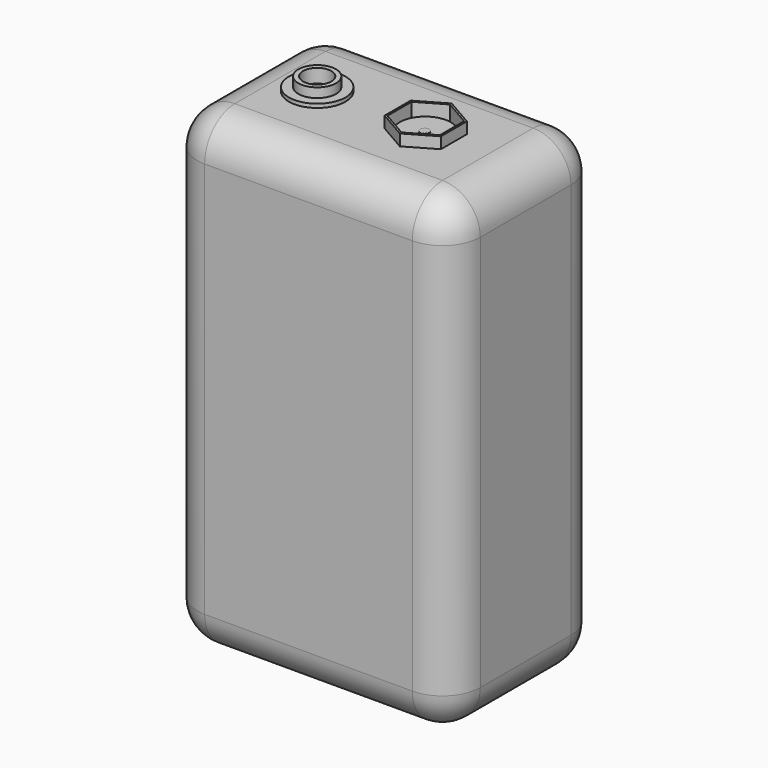
from build123d import *

# Parameters (mm, degrees)
F0_W      = 38.1
F0_H      = 63.5
F1_DEPTH  = 25.4
F2_R      = 5.08
F3_R      = 3.81
F4_DEPTH  = 0.508
F5_R      = 2.54
F6_DEPTH  = 1.27
F7_R      = 1.905
F8_DEPTH  = 1.8542
F10_DEPTH = 1.524
F13_DEPTH = 2.286
F14_R     = 3.429
F15_DEPTH = 0.5842
F16_R     = 0.635
F17_DEPTH = 0.0254
F18_R     = 0.635
F19_DEPTH = 0.254
F20_R     = 0.381
F21_DEPTH = 3.8354


with BuildPart() as f1:
    # F0 (on Front) → F1 (new body)
    with BuildSketch(Plane.XZ):
        Rectangle(F0_W, F0_H)
    extrude(amount=F1_DEPTH)

    # F2
    f2_edges = [f1.edges().sort_by_distance(p)[0] for p in [
        (19.05, -25.4, 0),
        (0, -25.4, 31.75),
        (-19.05, -25.4, 0),
        (0, -25.4, -31.75),
        (19.05, -12.7, -31.75),
        (19.05, -12.7, 31.75),
        (19.05, 0, 0),
        (0, 0, 31.75),
        (-19.05, 0, 0),
        (0, 0, -31.75),
        (-19.05, -12.7, 31.75),
        (-19.05, -12.7, -31.75),
    ]]
    fillet(f2_edges, radius=F2_R)

    # F3 (on face) → F4 (join)
    with BuildSketch(Plane.XY.offset(31.75)):
        with Locations((-8.9868323129, -12.7)):
            Circle(F3_R)
    extrude(amount=F4_DEPTH)

    # F5 (on face) → F6 (join)
    with BuildSketch(Plane.XY.offset(32.258)):
        with Locations((-8.9868323129, -12.7)):
            Circle(F5_R)
    extrude(amount=F6_DEPTH)

    # F7 (on face) → F8 (cut, symmetric)
    with BuildSketch(Plane.XY.offset(33.528)):
        with Locations((-8.9868323129, -12.7)):
            Circle(F7_R)
    extrude(amount=F8_DEPTH, both=True, mode=Mode.SUBTRACT)

    # F9 (on face) → F10 (join)
    with BuildSketch(Plane.XY.offset(31.75)):
        Polygon((9.4006182914, -14.8837988746), (9.4006182914, -10.5162011254), (5.6181676871, -8.3324022508), (1.8357170827, -10.5162011254), (1.8357170827, -14.8837988746), (5.6181676871, -17.0675977492), align=None)
    extrude(amount=F10_DEPTH)

    # F12 (on face) → F13 (cut)
    with BuildSketch(Plane.XY.offset(33.274)):
        Polygon((9.1466182914, -10.6628480938), (5.6181676871, -8.6256961876), (2.0897170827, -10.6628480938), (2.0897170827, -14.7371519062), (5.6181676871, -16.7743038124), (9.1466182914, -14.7371519062), align=None)
    extrude(amount=-F13_DEPTH, mode=Mode.SUBTRACT)


with BuildPart() as f15:
    # F14 (on face) → F15 (new body)
    with BuildSketch(Plane.XY.offset(31.75)):
        with Locations((5.6070124581, -12.7833363355)):
            Circle(F14_R)
    extrude(amount=-F15_DEPTH)


with BuildPart() as f17:
    # F16 (on face) → F17 (new body)
    with BuildSketch(Plane.XY.offset(31.75)):
        with Locations((5.5094454437, -12.7416318282)):
            Circle(F16_R)
    extrude(amount=F17_DEPTH)


with BuildPart() as f19:
    # F18 (on face) → F19 (new body)
    with BuildSketch(Plane.XY.offset(31.75)):
        with Locations((-8.9868323129, -12.7)):
            Circle(F18_R)
    extrude(amount=F19_DEPTH)

    # F20 (on face) → F21 (cut)
    with BuildSketch(Plane.XY.offset(32.004)):
        with Locations((-8.9868323129, -12.7)):
            Circle(F20_R)
    extrude(amount=-F21_DEPTH, mode=Mode.SUBTRACT)


solid = Compound([f1.part, f15.part, f17.part, f19.part])
